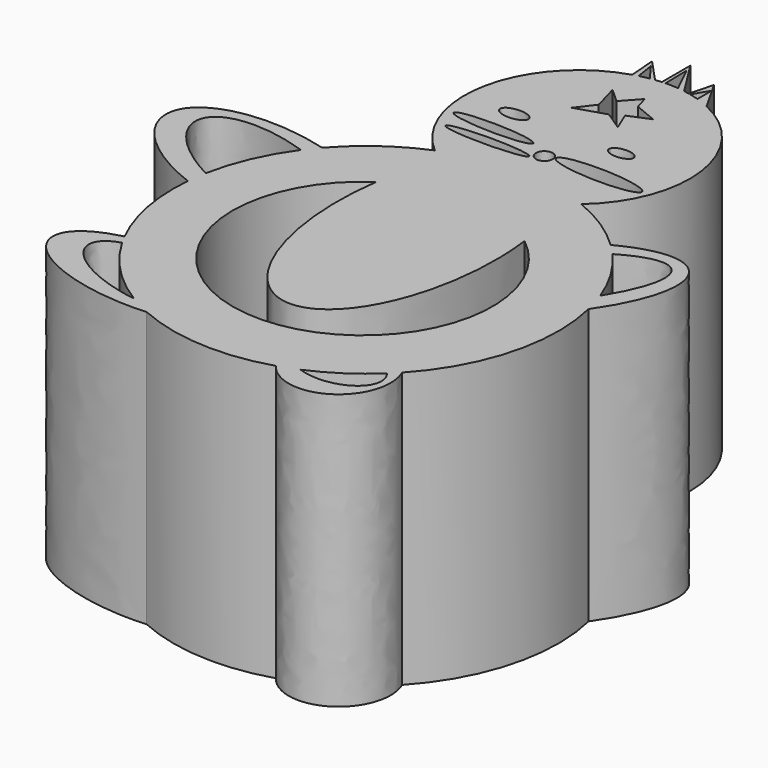
from build123d import *

# Parameters (mm, degrees)
F0_R     = 10.0785054584
F0_R_2   = 0.7726547986
F1_DEPTH = 25.4


# Not quite as in the source:
# - ends of sketch curves that miss each other by under 0.0002 mm in the source are joined


with BuildPart() as f1:
    # F0 (on Top) → F1 (new body)
    with BuildSketch(Plane.XY):
        with BuildLine():
            add(Edge.make_bspline(
                [(-50.0180964614, 28.8197003624), (-57.2975115577, 31.3487862827), (-58.6232181907, 28.2901978298), (-59.9489248237, 25.231609377), (-53.106087556, 21.6952780586)],
                knots=[1.7344668149, 1.7344668149, 1.7344668149, 3.1398513289, 3.1398513289, 4.545235843, 4.545235843, 4.545235843], degree=2, weights=[1, 0.7631050179, 1, 0.7631050179, 1]))
            ThreePointArc((-50.0180964614, 28.8197003624), (-49.5398823331, 29.4473185267), (-49.0343167088, 30.0531210625))
            add(Edge.make_bspline(
                [(-49.0343167088, 30.0531210625), (-58.9158228988, 32.7987351352), (-60.8866187286, 28.1822837461), (-62.8574145584, 23.5658323569), (-53.352182829, 19.9388216781)],
                knots=[1.6113627075, 1.6113627075, 1.6113627075, 3.0865508755, 3.0865508755, 4.5617390434, 4.5617390434, 4.5617390434], degree=2, weights=[1, 0.7400887, 1, 0.7400887, 1]))
            ThreePointArc((-53.352182829, 19.9388216781), (-53.2510312996, 20.8201177091), (-53.106087556, 21.6952780586))
        make_face()
        with BuildLine():
            ThreePointArc((-49.0343167088, 30.0531210625), (-49.5398823331, 29.4473185267), (-50.0180964614, 28.8197003624))
            ThreePointArc((-50.0180964614, 28.8197003624), (-51.9554128243, 25.427969163), (-53.106087556, 21.6952780586))
            ThreePointArc((-53.106087556, 21.6952780586), (-53.2510312996, 20.8201177091), (-53.352182829, 19.9388216781))
            ThreePointArc((-53.352182829, 19.9388216781), (-53.1054689981, 15.0033563173), (-51.5110108292, 10.3260291757))
            ThreePointArc((-51.5110108292, 10.3260291757), (-51.280508632, 9.8852244586), (-51.0377759492, 9.451034516))
            ThreePointArc((-51.0377759492, 9.451034516), (-48.3787694683, 5.9376819562), (-44.9380593764, 3.1853237423))
            ThreePointArc((-44.9380593764, 3.1853237423), (-43.9342610942, 2.613095927), (-42.8954439712, 2.1072158532))
            ThreePointArc((-42.8954439712, 2.1072158532), (-36.6982327212, 0.5877050753), (-30.3633878968, 1.3519572135))
            ThreePointArc((-30.3633878968, 1.3519572135), (-29.4684173588, 1.6553834073), (-28.5908161665, 2.0058914187))
            ThreePointArc((-28.5908161665, 2.0058914187), (-25.8280594304, 3.4968056801), (-23.3702871248, 5.4500095639))
            ThreePointArc((-23.3702871248, 5.4500095639), (-22.977856737, 5.8345656337), (-22.5974852794, 6.2310533816))
            ThreePointArc((-22.5974852794, 6.2310533816), (-18.4333953632, 13.7646746594), (-18.2923616242, 22.3713699526))
            ThreePointArc((-18.2923616242, 22.3713699526), (-18.5820570111, 23.4620905143), (-18.9403054317, 24.5322553755))
            ThreePointArc((-18.9403054317, 24.5322553755), (-20.3641292785, 27.4997757708), (-22.3101148735, 30.1543174841))
            ThreePointArc((-22.3101148735, 30.1543174841), (-22.7957304511, 30.6805123661), (-23.3021210637, 31.1867456034))
            ThreePointArc((-23.3021210637, 31.1867456034), (-25.9482355577, 33.283649081), (-28.9427655928, 34.8430451111))
            ThreePointArc((-28.9427655928, 34.8430451111), (-25.3977045999, 44.3102382619), (-31.4318132237, 52.4210173068))
            ThreePointArc((-31.4318132237, 52.4210173068), (-32.0373954884, 52.6778175418), (-32.6577872038, 52.8964276046))
            ThreePointArc((-32.6577872038, 52.8964276046), (-33.0851112648, 53.0223468137), (-33.517364649, 53.1301360167))
            ThreePointArc((-33.517364649, 53.1301360167), (-33.6017594974, 53.14893749), (-33.6863054157, 53.1670475296))
            ThreePointArc((-33.6863054157, 53.1670475296), (-33.9302645044, 53.2152700375), (-34.1752911752, 53.257736233))
            ThreePointArc((-34.1752911752, 53.257736233), (-34.4871149048, 53.3032446145), (-34.8001573646, 53.3394312076))
            ThreePointArc((-34.8001573646, 53.3394312076), (-35.2387913564, 53.3743052487), (-35.6784971845, 53.3908812059))
            ThreePointArc((-35.6784971845, 53.3908812059), (-35.8349745403, 53.3880712068), (-35.99139309, 53.3829432177))
            ThreePointArc((-35.99139309, 53.3829432177), (-36.1540493789, 53.3751479329), (-36.3165661693, 53.3648461076))
            ThreePointArc((-36.3165661693, 53.3648461076), (-36.6068663985, 53.3401682996), (-36.8963756174, 53.3074937009))
            ThreePointArc((-36.8963756174, 53.3074937009), (-37.1124002353, 53.2778219809), (-37.3277663495, 53.2436974533))
            ThreePointArc((-37.3277663495, 53.2436974533), (-37.7755052177, 53.1580322854), (-38.2191310496, 53.0531288233))
            ThreePointArc((-38.2191310496, 53.0531288233), (-38.457404707, 52.9883450288), (-38.6940989785, 52.9180094213))
            ThreePointArc((-38.6940989785, 52.9180094213), (-45.91294383, 44.9596494894), (-42.4272827417, 34.7961175947))
            ThreePointArc((-42.4272827417, 34.7961175947), (-46.0053988989, 32.8071382816), (-49.0343167088, 30.0531210625))
        make_face()
        with BuildLine():
            ThreePointArc((-40.1754545674, 33.3235095623), (-38.0178952671, 32.5534974638), (-35.7450652159, 32.266749623))
            ThreePointArc((-35.7450652159, 32.266749623), (-33.4705135315, 32.539157888), (-31.3081785908, 33.2955303043))
            ThreePointArc((-31.3081785908, 33.2955303043), (-20.2401657347, 16.065589316), (-35.8379356915, 2.7960246127))
            ThreePointArc((-35.8379356915, 2.7960246127), (-51.3517644926, 16.1636306426), (-40.1754545674, 33.3235095623))
        make_face(mode=Mode.SUBTRACT)
        with Locations((-35.5670807588, 42.828359423)):
            Circle(F0_R, mode=Mode.SUBTRACT)
        with BuildLine():
            ThreePointArc((-51.0377759492, 9.451034516), (-51.280508632, 9.8852244586), (-51.5110108292, 10.3260291757))
            add(Edge.make_bspline(
                [(-51.5110108292, 10.3260291757), (-58.27393887, 8.6796410588), (-54.5247475311, 5.1031028887), (-50.7755561922, 1.5265647186), (-42.8954439712, 2.1072158532)],
                knots=[2.2296629378, 2.2296629378, 2.2296629378, 3.6509124512, 3.6509124512, 5.0721619646, 5.0721619646, 5.0721619646], degree=2, weights=[1, 0.7579544905, 1, 0.7579544905, 1]))
            ThreePointArc((-42.8954439712, 2.1072158532), (-43.9342610942, 2.613095927), (-44.9380593764, 3.1853237423))
            add(Edge.make_bspline(
                [(-51.0377759492, 9.451034516), (-63.3998983234, 5.6216599189), (-44.9380593764, 3.1853237423)],
                knots=[2.5213368346, 2.5213368346, 2.5213368346, 4.9609070517, 4.9609070517, 4.9609070517], degree=2, weights=[1, 0.3438475428, 1]))
        make_face()
        with BuildLine():
            Line((-38.8921536505, 55.4570183158), (-38.6940989785, 52.9180094213))
            ThreePointArc((-38.6940989785, 52.9180094213), (-38.457404707, 52.9883450288), (-38.2191310496, 53.0531288233))
            Line((-38.2191310496, 53.0531288233), (-38.4829491377, 54.8071041703))
            Line((-38.4829491377, 54.8071041703), (-37.3277663495, 53.2436974533))
            ThreePointArc((-37.3277663495, 53.2436974533), (-37.1124002353, 53.2778219809), (-36.8963756174, 53.3074937009))
            Line((-36.8963756174, 53.3074937009), (-38.8921536505, 55.4570183158))
        make_face()
        with BuildLine():
            ThreePointArc((-28.5908161665, 2.0058914187), (-29.4684173588, 1.6553834073), (-30.3633878968, 1.3519572135))
            add(Edge.make_bspline(
                [(-30.3633878968, 1.3519572135), (-27.965591922, -1.791721016), (-24.4898843488, 0.3919673893), (-21.0141767755, 2.5756557946), (-22.5974852794, 6.2310533816)],
                knots=[2.889066059, 2.889066059, 2.889066059, 4.3424240407, 4.3424240407, 5.7957820224, 5.7957820224, 5.7957820224], degree=2, weights=[1, 0.7473849691, 1, 0.7473849691, 1]))
            ThreePointArc((-22.5974852794, 6.2310533816), (-22.977856737, 5.8345656337), (-23.3702871248, 5.4500095639))
            add(Edge.make_bspline(
                [(-28.5908161665, 2.0058914187), (-17.2479026501, -2.1550631546), (-23.3702871248, 5.4500095639)],
                knots=[4.2093542263, 4.2093542263, 4.2093542263, 6.7757546269, 6.7757546269, 6.7757546269], degree=2, weights=[1, 0.283647904, 1]))
        make_face()
        with BuildLine():
            Line((-36.3165661693, 56.6605627537), (-36.3165661693, 53.3648461076))
            ThreePointArc((-36.3165661693, 53.3648461076), (-36.1540493789, 53.3751479329), (-35.99139309, 53.3829432177))
            Line((-35.99139309, 53.3829432177), (-36.0340364277, 55.8662228286))
            Line((-36.0340364277, 55.8662228286), (-34.8001573646, 53.3394312076))
            ThreePointArc((-34.8001573646, 53.3394312076), (-34.4871149048, 53.3032446145), (-34.1752911752, 53.257736233))
            Line((-34.1752911752, 53.257736233), (-36.3165661693, 56.6605627537))
        make_face()
        with BuildLine():
            ThreePointArc((-18.9403054317, 24.5322553755), (-18.5820570111, 23.4620905143), (-18.2923616242, 22.3713699526))
            add(Edge.make_bspline(
                [(-18.2923616242, 22.3713699526), (-5.6099736512, 40.5672382573), (-23.3021210637, 31.1867456034)],
                knots=[5.0525203643, 5.0525203643, 5.0525203643, 7.246140576, 7.246140576, 7.246140576], degree=2, weights=[1, 0.456436666, 1]))
            ThreePointArc((-23.3021210637, 31.1867456034), (-22.7957304511, 30.6805123661), (-22.3101148735, 30.1543174841))
            add(Edge.make_bspline(
                [(-18.9403054317, 24.5322553755), (-11.291213279, 36.7310525289), (-22.3101148735, 30.1543174841)],
                knots=[5.1975250581, 5.1975250581, 5.1975250581, 7.160862441, 7.160862441, 7.160862441], degree=2, weights=[1, 0.555635928, 1]))
        make_face()
        with BuildLine():
            Line((-33.0910608172, 55.3607344627), (-33.6863054157, 53.1670475296))
            ThreePointArc((-33.6863054157, 53.1670475296), (-33.6017594974, 53.14893749), (-33.517364649, 53.1301360167))
            Line((-33.517364649, 53.1301360167), (-32.6577872038, 54.5663945377))
            Line((-32.6577872038, 54.5663945377), (-32.6577872038, 52.8964276046))
            ThreePointArc((-32.6577872038, 52.8964276046), (-32.0373954884, 52.6778175418), (-31.4318132237, 52.4210173068))
            Line((-31.4318132237, 52.4210173068), (-33.0910608172, 55.3607344627))
        make_face()
        with BuildLine():
            ThreePointArc((-31.3081785908, 33.2955303043), (-33.4705135315, 32.539157888), (-35.7450652159, 32.266749623))
            ThreePointArc((-35.7450652159, 32.266749623), (-38.0178952671, 32.5534974638), (-40.1754545674, 33.3235095623))
            ThreePointArc((-40.1754545674, 33.3235095623), (-51.3517644926, 16.1636306426), (-35.8379356915, 2.7960246127))
            ThreePointArc((-35.8379356915, 2.7960246127), (-20.2401657347, 16.065589316), (-31.3081785908, 33.2955303043))
        make_face()
        with BuildLine():
            ThreePointArc((-42.6517156255, 28.3089399398), (-41.2780913199, 29.10675124), (-39.811138088, 29.716172949))
            add(Edge.make_bspline(
                [(-39.811138088, 29.716172949), (-44.2325567375, 13.8247773653), (-35.6994618661, 13.5522226968), (-27.1663669947, 13.2796680283), (-31.3717468344, 29.4466112577)],
                knots=[4.1677682594, 4.1677682594, 4.1677682594, 6.2685150493, 6.2685150493, 8.3692618392, 8.3692618392, 8.3692618392], degree=2, weights=[1, 0.4972471218, 1, 0.4972471218, 1]))
            ThreePointArc((-31.3717468344, 29.4466112577), (-29.8950207475, 28.7148058545), (-28.5324694133, 27.7875987873))
            ThreePointArc((-28.5324694133, 27.7875987873), (-36.3929905001, 6.3579122365), (-42.6517156255, 28.3089399398))
        make_face(mode=Mode.SUBTRACT)
        with BuildLine():
            add(Edge.make_bspline(
                [(-39.811138088, 29.716172949), (-44.2325567375, 13.8247773653), (-35.6994618661, 13.5522226968), (-27.1663669947, 13.2796680283), (-31.3717468344, 29.4466112577)],
                knots=[4.1677682594, 4.1677682594, 4.1677682594, 6.2685150493, 6.2685150493, 8.3692618392, 8.3692618392, 8.3692618392], degree=2, weights=[1, 0.4972471218, 1, 0.4972471218, 1]))
            ThreePointArc((-39.811138088, 29.716172949), (-41.2780913199, 29.10675124), (-42.6517156255, 28.3089399398))
            add(Edge.make_bspline(
                [(-42.6517156255, 28.3089399398), (-45.345902533, 9.9359036694), (-35.7629848612, 9.5820625884), (-26.1800671894, 9.2282215074), (-28.5324694133, 27.7875987873)],
                knots=[4.4274522653, 4.4274522653, 4.4274522653, 6.2647020613, 6.2647020613, 8.1019518573, 8.1019518573, 8.1019518573], degree=2, weights=[1, 0.6069136169, 1, 0.6069136169, 1]))
            ThreePointArc((-28.5324694133, 27.7875987873), (-29.8950207475, 28.7148058545), (-31.3717468344, 29.4466112577))
        make_face()
        with Locations((-35.5670807588, 42.828359423)):
            Circle(F0_R)
        with BuildLine():
            add(Edge.make_bspline(
                [(-36.5413166583, 38.3234322071), (-36.5413166583, 39.1777903129), (-42.3355195671, 38.75061126), (-48.129722476, 38.3234322071), (-42.3355195671, 37.8962531542), (-36.5413166583, 37.4690741013), (-36.5413166583, 38.3234322071)],
                knots=[0, 0, 0, 2.0943951024, 2.0943951024, 4.1887902048, 4.1887902048, 6.2831853072, 6.2831853072, 6.2831853072], degree=2, weights=[1, 0.5, 1, 0.5, 1, 0.5, 1]))
        make_face(mode=Mode.SUBTRACT)
        with BuildLine():
            add(Edge.make_bspline(
                [(-37.5765897334, 40.0711521506), (-37.5496060824, 41.0785421219), (-43.1736253786, 40.7251290722), (-48.7976446748, 40.3717160225), (-43.2006090296, 39.7177391009), (-37.6035733843, 39.0637621794), (-37.5765897334, 40.0711521506)],
                knots=[0, 0, 0, 2.0943951024, 2.0943951024, 4.1887902048, 4.1887902048, 6.2831853072, 6.2831853072, 6.2831853072], degree=2, weights=[1, 0.5, 1, 0.5, 1, 0.5, 1]))
        make_face(mode=Mode.SUBTRACT)
        with BuildLine():
            add(Edge.make_bspline(
                [(-40.1991009712, 42.828359423), (-40.1991009712, 43.9732546132), (-42.1727709472, 43.4008070181), (-44.1464409232, 42.828359423), (-42.1727709472, 42.2559118279), (-40.1991009712, 41.6834642328), (-40.1991009712, 42.828359423)],
                knots=[0, 0, 0, 2.0943951024, 2.0943951024, 4.1887902048, 4.1887902048, 6.2831853072, 6.2831853072, 6.2831853072], degree=2, weights=[1, 0.5, 1, 0.5, 1, 0.5, 1]))
        make_face(mode=Mode.SUBTRACT)
        with Locations((-35.7072949409, 39.0425398946)):
            Circle(F0_R_2, mode=Mode.SUBTRACT)
        with BuildLine():
            add(Edge.make_bspline(
                [(-26.718609035, 39.0541218221), (-26.6681576645, 40.4621885374), (-32.7954675319, 39.97679433), (-38.9227773994, 39.4914001226), (-32.8459189025, 38.5687276147), (-26.7690604056, 37.6460551068), (-26.718609035, 39.0541218221)],
                knots=[0, 0, 0, 2.0943951024, 2.0943951024, 4.1887902048, 4.1887902048, 6.2831853072, 6.2831853072, 6.2831853072], degree=2, weights=[1, 0.5, 1, 0.5, 1, 0.5, 1]))
        make_face(mode=Mode.SUBTRACT)
        Polygon((-37.005212158, 48.9953197539), (-35.6241986156, 50.5217015743), (-35.2607704699, 49.2860600352), (-33.1645212472, 48.4271711887), (-35.1154021919, 47.6143062115), (-34.3885533512, 45.8698645234), (-36.1329913139, 47.0328256488), (-38.8950183988, 46.1606048048), (-37.6593731344, 47.7596744895), (-38.3355605541, 50.1989695397), align=None, mode=Mode.SUBTRACT)
        with BuildLine():
            add(Edge.make_bspline(
                [(-30.4895397276, 42.828359423), (-30.4895397276, 43.8939900952), (-32.1909794584, 43.3611747591), (-33.8924191892, 42.828359423), (-32.1909794584, 42.2955440869), (-30.4895397276, 41.7627287508), (-30.4895397276, 42.828359423)],
                knots=[0, 0, 0, 2.0943951024, 2.0943951024, 4.1887902048, 4.1887902048, 6.2831853072, 6.2831853072, 6.2831853072], degree=2, weights=[1, 0.5, 1, 0.5, 1, 0.5, 1]))
        make_face(mode=Mode.SUBTRACT)
    extrude(amount=F1_DEPTH)


solid = f1.part
